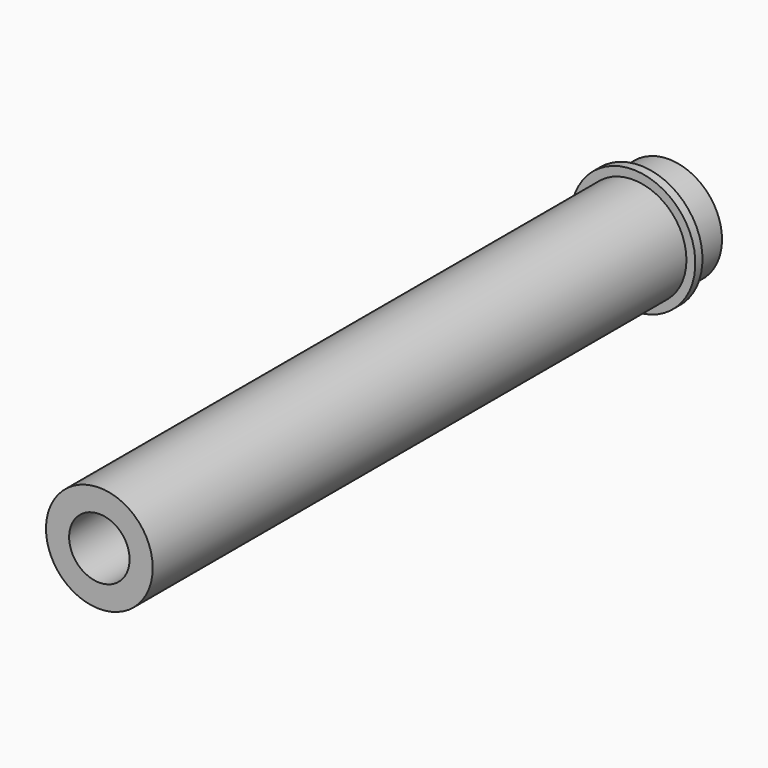
from build123d import *

# Parameters (mm, degrees)
F0_R     = 6
F1_DEPTH = 75
F2_R     = 7
F2_R_2   = 6
F3_DEPTH = 1
F4_R     = 6
F5_DEPTH = 4
F7_D     = 6.8
F7_DEPTH = 15
F7_TIP   = 2.0429261047


with BuildPart() as f1:
    # F0 (on Front) → F1 (new body)
    with BuildSketch(Plane.XZ):
        Circle(F0_R)
    extrude(amount=F1_DEPTH)

    # F2 (on face) → F3 (join)
    with BuildSketch(Plane(origin=(0, 0, 0), x_dir=(-1, 0, 0), z_dir=(0, 1, 0))):
        Circle(F2_R)
        Circle(F2_R_2, mode=Mode.SUBTRACT)
        Circle(F2_R_2)
    extrude(amount=F3_DEPTH)

    # F4 (on face) → F5 (join)
    with BuildSketch(Plane(origin=(0, 1, 0), x_dir=(-1, 0, 0), z_dir=(0, 1, 0))):
        Circle(F4_R)
    extrude(amount=F5_DEPTH)

    # F7
    with Locations(Plane.XZ.offset(75)):
        with Locations((0, 0)):
            Hole(F7_D / 2, depth=F7_DEPTH)
            with Locations((0, 0, -(F7_DEPTH + F7_TIP / 2))):  # 118° drill point
                Cone(0, F7_D / 2, F7_TIP, mode=Mode.SUBTRACT)


solid = f1.part
